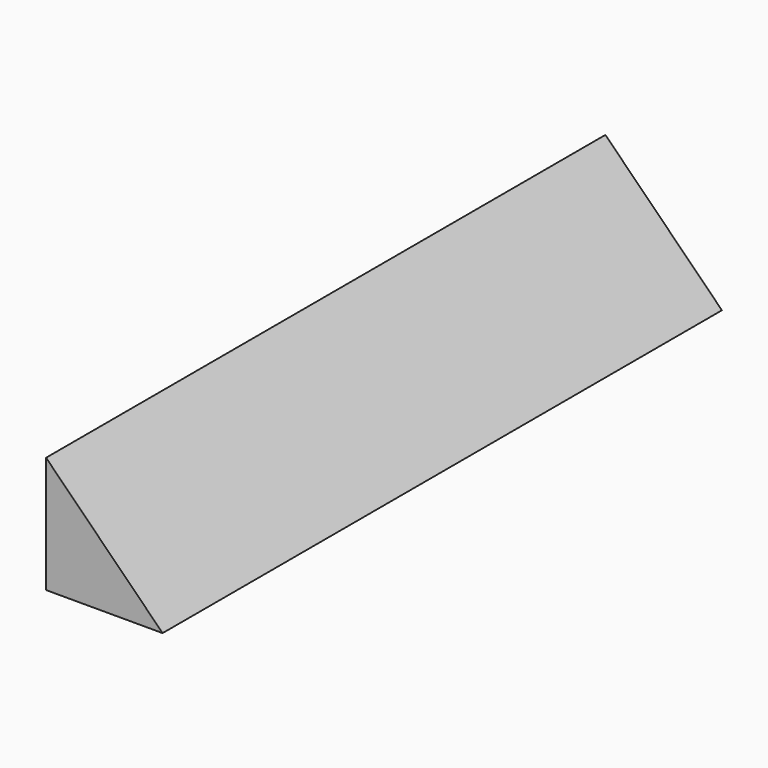
from build123d import *

# Parameters (mm, degrees)
F0_W     = 12.7
F0_H     = 12.7
F1_DEPTH = 76.2
F2_SIZE  = 12.69999


# Not quite as in the source:
# - a fillet or chamfer is up to 0.001 mm smaller than in the source, because OpenCascade refuses the exact size


with BuildPart() as f1:
    # F0 (on Front) → F1 (new body)
    with BuildSketch(Plane.XZ):
        with Locations((-194.5890816092, 6.35)):
            Rectangle(F0_W, F0_H)
    extrude(amount=F1_DEPTH)

    # F2 (size 12.7 in the source; OpenCascade refuses exactly that, so slightly less here)
    f2_edges = [f1.edges().sort_by_distance(p)[0] for p in [
        (-188.239082, -38.1, 12.7),
    ]]
    chamfer(f2_edges, length=F2_SIZE)


solid = f1.part
